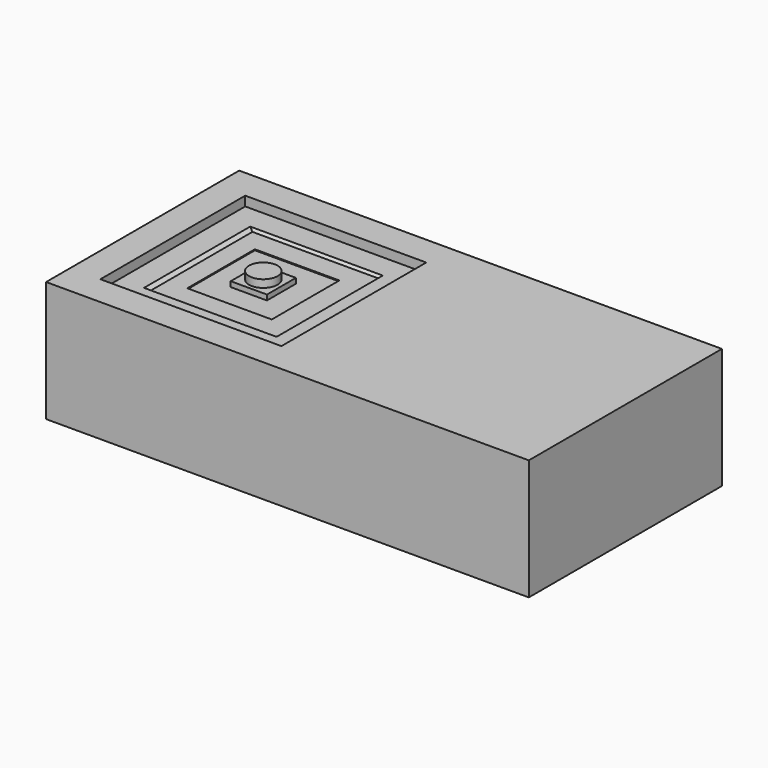
from build123d import *

# Parameters (mm, degrees)
F0_W        = 50.8
F0_H        = 25.4
F1_DEPTH    = 12.7
F2_W        = 19.05
F2_H        = 19.05
F2_W_2      = 13.97
F2_H_2      = 13.97
F2_W_3      = 8.89
F2_H_3      = 8.89
F2_W_4      = 3.81
F2_H_4      = 3.81
F3_DEPTH    = 1
F4_DEPTH    = 1.25
F5_DEPTH    = 1.35
F6_SIZE2    = 0.24999
F6_SIZE     = 0.24999
F7_T4_DEPTH = 16.0483871792
F8_W        = 3.81
F8_H        = 3.81
F8_R        = 1.5
F9_DEPTH    = 0.8


# Not quite as in the source:
# - a fillet or chamfer that OpenCascade refuses, or shapes differently, is made with other operations: its cross-section is extruded or revolved along the edge and cut away or added
# - a fillet or chamfer is up to 0.001 mm smaller than in the source, because OpenCascade refuses the exact size


with BuildPart() as f1:
    # F0 (on Top) → F1 (new body)
    with BuildSketch(Plane.XY):
        Rectangle(F0_W, F0_H)
    extrude(amount=F1_DEPTH)

    # F2 (on face) → F3 (cut)
    with BuildSketch(Plane.XY.offset(12.7)):
        with Locations((-12.7, 0)):
            Rectangle(F2_W, F2_H)
        with Locations((-12.7, 0)):
            Rectangle(F2_W_2, F2_H_2, mode=Mode.SUBTRACT)
        with Locations((-12.7, 0)):
            Rectangle(F2_W_2, F2_H_2)
        with Locations((-12.7, 0)):
            Rectangle(F2_W_3, F2_H_3, mode=Mode.SUBTRACT)
        with Locations((-12.7, 0)):
            Rectangle(F2_W_3, F2_H_3)
        with Locations((-12.7, 0)):
            Rectangle(F2_W_4, F2_H_4, mode=Mode.SUBTRACT)
    extrude(amount=-F3_DEPTH, mode=Mode.SUBTRACT)

    # F2 (on face) → F4 (cut)
    with BuildSketch(Plane.XY.offset(12.7)):
        with Locations((-12.7, 0)):
            Rectangle(F2_W_2, F2_H_2)
        with Locations((-12.7, 0)):
            Rectangle(F2_W_3, F2_H_3, mode=Mode.SUBTRACT)
    extrude(amount=-F4_DEPTH, mode=Mode.SUBTRACT)

    # F2 (on face) → F5 (cut)
    with BuildSketch(Plane.XY.offset(12.7)):
        with Locations((-12.7, 0)):
            Rectangle(F2_W_3, F2_H_3)
        with Locations((-12.7, 0)):
            Rectangle(F2_W_4, F2_H_4, mode=Mode.SUBTRACT)
    extrude(amount=-F5_DEPTH, mode=Mode.SUBTRACT)

    # F6 (size 0.25 and 0.25 in the source; OpenCascade refuses exactly that, so slightly less here)
    f6_edges = [f1.edges().sort_by_distance(p)[0] for p in [
        (-12.7, 6.985, 11.45),
    ]]
    chamfer(f6_edges, length=F6_SIZE, length2=F6_SIZE2)

    # F7: chamfer of 0.45 x 0.2598076211 on 1 edges, made by hand


with BuildPart() as f7_tool2:
    # F7_s3 → F7_t4 (new body)
    with BuildSketch(Plane.XZ.offset(-7.8991985896)):
        Polygon((-19.235, 11.45), (-19.685, 11.7098076211), (-19.685, 11.45), align=None)
    extrude(amount=F7_T4_DEPTH)

    split(bisect_by=Plane.XY.offset(11.7), keep=Keep.BOTTOM)


with BuildPart() as f1_1:
    add(f1.part)

    # F7_t1: union F7_tool2
    add(f7_tool2.part)

    # F8 (on face) → F9 (cut)
    with BuildSketch(Plane.XY.offset(12.7)):
        with Locations((-12.7, 0)):
            Rectangle(F8_W, F8_H)
        with Locations((-12.7, 0)):
            Circle(F8_R, mode=Mode.SUBTRACT)
    extrude(amount=-F9_DEPTH, mode=Mode.SUBTRACT)


solid = f1_1.part
